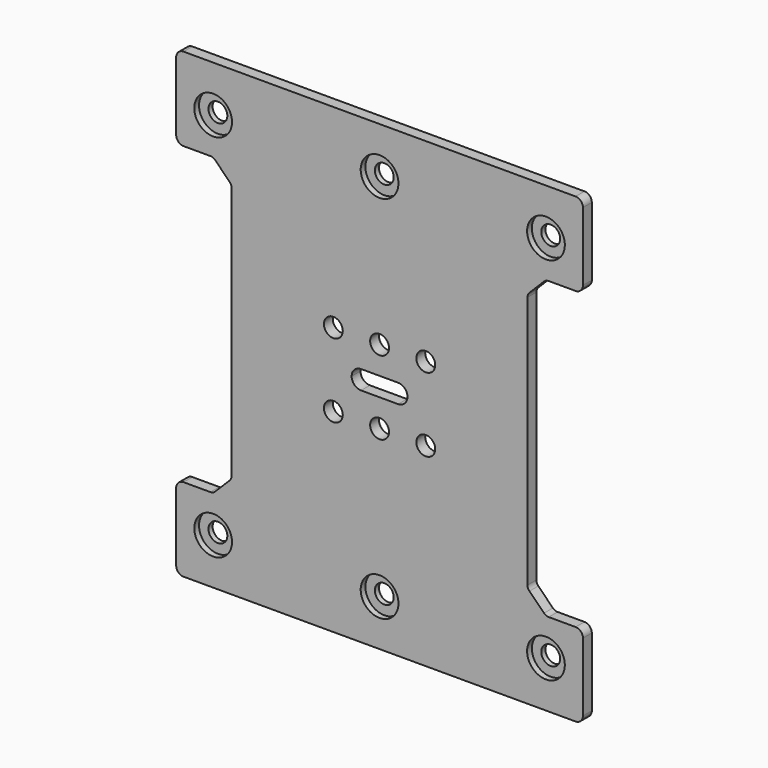
from build123d import *

# Parameters (mm, degrees)
F1_DEPTH       = 3
F2_D           = 5.1
F2_DEPTH       = 34.5
F2_TIP         = 1.5321945785
F3_D           = 5.1
F3_DEPTH       = 34.5
F3_CBORE_D     = 10.2
F3_CBORE_DEPTH = 1.6
F3_TIP         = 1.5321945785
F5_D           = 5.1
F5_DEPTH       = 34.5
F5_TIP         = 1.5321945785
F6_D           = 5.1
F6_DEPTH       = 34.5
F6_CBORE_D     = 10.2
F6_CBORE_DEPTH = 1.6
F6_TIP         = 1.5321945785


# Not quite as in the source:
# - a feature names something its author has since deleted; it is built from what else it names


with BuildPart() as f1:
    # F0 (on Front) → F1 (new body)
    with BuildSketch(Plane.XZ):
        with BuildLine():
            Line((-157.7735108339, 88.9936834574), (-210.7735108339, 88.9936834574))
            ThreePointArc((-210.7735108339, 88.9936834574), (-212.1877243962, 88.4078970197), (-212.7735108339, 86.9936834574))
            Line((-212.7735108339, 86.9936834574), (-212.7735108339, 68.4936834574))
            ThreePointArc((-212.7735108339, 68.4936834574), (-212.1877243962, 67.079469895), (-210.7735108339, 66.4936834574))
            Line((-210.7735108339, 66.4936834574), (-203.5195108339, 66.4936834574))
            ThreePointArc((-203.5195108339, 66.4936834574), (-202.8306806556, 66.3566666159), (-202.2467186277, 65.9664756635))
            Line((-202.2467186277, 65.9664756635), (-198.3007186277, 62.0204756635))
            ThreePointArc((-198.3007186277, 62.0204756635), (-197.9105276754, 61.4365136356), (-197.7735108339, 60.7476834574))
            Line((-197.7735108339, 60.7476834574), (-197.7735108339, 26.4936834574))
            Line((-197.7735108339, 26.4936834574), (-165.3235108339, 26.4936834574))
            ThreePointArc((-165.3235108339, 26.4936834574), (-164.5766331259, 28.2968057494), (-162.7735108339, 29.0436834574))
            Line((-162.7735108339, 29.0436834574), (-157.7735108339, 29.0436834574))
            Line((-157.7735108339, 29.0436834574), (-157.7735108339, 88.9936834574))
        make_face()
    extrude(amount=-F1_DEPTH)

    # F2
    with Locations(Plane.XZ):
        with Locations((-170.2735108339, 36.4936834574)):
            Hole(F2_D / 2, depth=F2_DEPTH)
            with Locations((0, 0, -(F2_DEPTH + F2_TIP / 2))):  # 118° drill point
                Cone(0, F2_D / 2, F2_TIP, mode=Mode.SUBTRACT)

    # F3
    with Locations(Plane.XZ):
        with Locations((-202.7735108339, 76.4936834574)):
            CounterBoreHole(F3_D / 2, F3_CBORE_D / 2, F3_CBORE_DEPTH, depth=F3_DEPTH)
            with Locations((0, 0, -(F3_DEPTH + F3_TIP / 2))):  # 118° drill point
                Cone(0, F3_D / 2, F3_TIP, mode=Mode.SUBTRACT)

    # F4: F1 across face


with BuildPart() as f1_1:
    add(f1.part)
    add(f1.part.mirror(Plane(origin=(-157.7735108339, 1.5, 59.0186834574), x_dir=(0, 1, 0), z_dir=(1, 0, 0))))

    # F5
    with Locations(Plane.XZ):
        with Locations((-157.7735108339, 36.4936834574)):
            Hole(F5_D / 2, depth=F5_DEPTH)
            with Locations((0, 0, -(F5_DEPTH + F5_TIP / 2))):  # 118° drill point
                Cone(0, F5_D / 2, F5_TIP, mode=Mode.SUBTRACT)

    # F6
    with Locations(Plane.XZ):
        with Locations((-157.7735108339, 76.4936834574)):
            CounterBoreHole(F6_D / 2, F6_CBORE_D / 2, F6_CBORE_DEPTH, depth=F6_DEPTH)
            with Locations((0, 0, -(F6_DEPTH + F6_TIP / 2))):  # 118° drill point
                Cone(0, F6_D / 2, F6_TIP, mode=Mode.SUBTRACT)

    # F7: F1 across face


with BuildPart() as f1_2:
    add(f1_1.part)
    add(f1_1.part.mirror(Plane(origin=(-181.5485108339, 1.5, 26.4936834574), x_dir=(1, 0, 0), z_dir=(0, 0, -1))))


solid = f1_2.part
